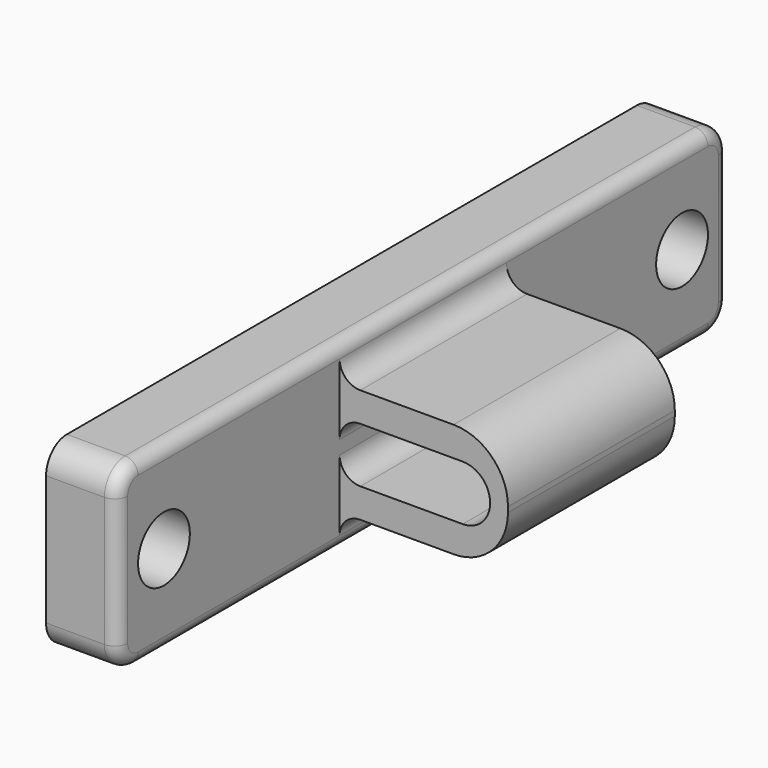
from build123d import *

# Parameters (mm, degrees)
F0_W     = 59
F0_H     = 14
F0_R     = 2.5
F0_W_2   = 16.1
F0_H_2   = 8.8
F1_DEPTH = 5.5
F2_DEPTH = 18.5
F3_R     = 4.2
F4_R     = 2
F5_R     = 1
F7_DEPTH = 25
F8_R     = 1.59999


# Not quite as in the source:
# - a fillet or chamfer is up to 0.001 mm smaller than in the source, because OpenCascade refuses the exact size


with BuildPart() as f1:
    # F0 (on Right) → F1 (new body)
    with BuildSketch(Plane.YZ):
        Rectangle(F0_W, F0_H)
        with Locations((-25, 0)):
            Circle(F0_R, mode=Mode.SUBTRACT)
        Rectangle(F0_W_2, F0_H_2, mode=Mode.SUBTRACT)
        with Locations((25, 0)):
            Circle(F0_R, mode=Mode.SUBTRACT)
    extrude(amount=F1_DEPTH)

    # F0 (on Right) → F2 (join)
    with BuildSketch(Plane.YZ):
        Rectangle(F0_W_2, F0_H_2)
        Circle(F0_R, mode=Mode.SUBTRACT)
        Circle(F0_R)
    extrude(amount=F2_DEPTH)

    # F3
    f3_edges = [f1.edges().sort_by_distance(p)[0] for p in [
        (18.5, 0, 4.4),
        (18.5, 0, -4.4),
    ]]
    fillet(f3_edges, radius=F3_R)

    # F4
    f4_edges = [f1.edges().sort_by_distance(p)[0] for p in [
        (2.75, 29.5, 7),
        (2.75, 29.5, -7),
        (2.75, -29.5, 7),
        (2.75, -29.5, -7),
    ]]
    fillet(f4_edges, radius=F4_R)

    # F5
    f5_edges = [f1.edges().sort_by_distance(p)[0] for p in [
        (5.5, 0, 7),
    ]]
    fillet(f5_edges, radius=F5_R)

    # F6 (on face) → F7 (cut)
    with BuildSketch(Plane.XZ.offset(8.05)):
        with BuildLine():
            Line((5.5, 2.125), (5.5, -2.125))
            Line((5.5, -2.125), (15, -2.125))
            ThreePointArc((15, -2.125), (17.125, 0), (15, 2.125))
            Line((15, 2.125), (5.5, 2.125))
        make_face()
    extrude(amount=-F7_DEPTH, mode=Mode.SUBTRACT)

    # F8 (radius 1.6 in the source; OpenCascade refuses exactly that, so slightly less here)
    f8_edges = [f1.edges().sort_by_distance(p)[0] for p in [
        (5.5, 0, 4.4),
        (5.5, 0, -4.4),
        (5.5, 0, -2.125),
        (5.5, 0, 2.125),
    ]]
    fillet(f8_edges, radius=F8_R)


solid = f1.part
